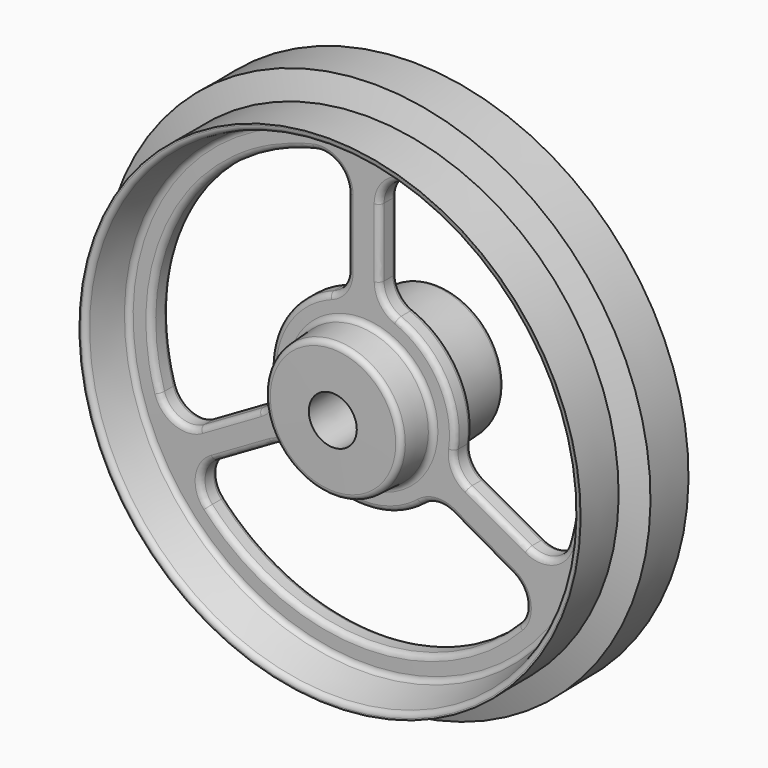
from build123d import *

# Parameters (mm, degrees)
F3_DEPTH = 43.6186672242
F4_R     = 2.54


with BuildPart() as f1:
    # F0 (on Right) → F1 (revolve)
    with BuildSketch(Plane.YZ):
        with BuildLine():
            Line((-17.1431349548, 28.9278083222), (-17.1431349548, 10.9819196094))
            Line((-17.1431349548, 10.9819196094), (43.1818650452, 10.9819196094))
            Line((43.1818650452, 10.9819196094), (43.1818650452, 28.867559352))
            ThreePointArc((43.1818650452, 28.867559352), (42.4756452655, 30.6250718281), (40.7496996094, 31.4052692856))
            Line((40.7496996094, 31.4052692856), (12.594030481, 32.601684317))
            ThreePointArc((12.594030481, 32.601684317), (10.8680848248, 33.3818817744), (10.1618650452, 35.1393942505))
            Line((10.1618650452, 35.1393942505), (10.1618650452, 115.7784299063))
            ThreePointArc((10.1618650452, 115.7784299063), (10.6173699596, 117.2298017531), (11.8205109018, 118.1606169002))
            Line((11.8205109018, 118.1606169002), (27.5388583799, 123.9760422684))
            ThreePointArc((27.5388583799, 123.9760422684), (28.7419993222, 124.9068574154), (29.1975042365, 126.3582292623))
            Line((29.1975042365, 126.3582292623), (29.1975042365, 127.2266535884))
            Line((29.1975042365, 127.2266535884), (6.9725042365, 127.2266535884))
            Line((6.9725042365, 127.2266535884), (2.6667747842, 115.951028812))
            Line((2.6667747842, 115.951028812), (-19.5582252158, 115.951028812))
            Line((-19.5582252158, 115.951028812), (-19.5582252158, 115.2566707518))
            ThreePointArc((-19.5582252158, 115.2566707518), (-19.0016386227, 113.6699536197), (-17.575806903, 112.7786266315))
            Line((-17.575806903, 112.7786266315), (-1.9805532676, 109.269557619))
            ThreePointArc((-1.9805532676, 109.269557619), (-0.5547215479, 108.3782306309), (0.0018650452, 106.7915134988))
            Line((0.0018650452, 106.7915134988), (0.0018650452, 34.8349003864))
            ThreePointArc((0.0018650452, 34.8349003864), (-0.6825103243, 33.1004675596), (-2.3668414357, 32.3006828484))
            Line((-2.3668414357, 32.3006828484), (-14.7744284739, 31.4620258603))
            ThreePointArc((-14.7744284739, 31.4620258603), (-16.4587595853, 30.662241149), (-17.1431349548, 28.9278083222))
        make_face()
    revolve(axis=Axis((0, -8.6872753461, -0.0663357208), (0, -0.9999708473, -0.0076357413)))

    # F2 (on Front) → F3 (cut, through all)
    with BuildSketch(Plane.XZ):
        with BuildLine():
            Line((-6.7658544631, 51.822418936), (-6.7658544631, 83.3901949943))
            ThreePointArc((-6.7658544631, 83.3901949943), (-11.5720090409, 93.33892378), (-22.3528157938, 95.7577110859))
            ThreePointArc((-22.3528157938, 95.7577110859), (-84.8589980062, 49.680358933), (-94.4432492338, -27.3799247713))
            ThreePointArc((-94.4432492338, -27.3799247713), (-86.9661995123, -35.6337295109), (-75.8589460274, -34.8210270811))
            Line((-75.8589460274, -34.8210270811), (-48.408480742, -18.8504932245))
            ThreePointArc((-48.408480742, -18.8504932245), (-43.3625739207, -13.4038718555), (-42.2241365486, -6.0669228754))
            ThreePointArc((-42.2241365486, -6.0669228754), (-36.7105113145, 21.7261045629), (-15.0000612074, 39.9334875039))
            ThreePointArc((-15.0000612074, 39.9334875039), (-9.0254144737, 44.5914291817), (-6.7658544631, 51.822418936))
        make_face()
        with BuildLine():
            ThreePointArc((23.8493413892, 95.3959984571), (12.9533792237, 93.0854213315), (8.0690974061, 83.0751990916))
            Line((8.0690974061, 83.0751990916), (8.0690974061, 51.3140057615))
            ThreePointArc((8.0690974061, 51.3140057615), (10.2381265661, 44.2155092188), (16.0043183773, 39.5417128325))
            ThreePointArc((16.0043183773, 39.5417128325), (37.0297436849, 21.1774253176), (42.1964618524, -6.2565060206))
            ThreePointArc((42.1964618524, -6.2565060206), (43.3372856677, -13.6718080208), (48.4641868849, -19.1493135334))
            Line((48.4641868849, -19.1493135334), (75.959996049, -34.8412705892))
            ThreePointArc((75.959996049, -34.8412705892), (87.0270006495, -35.5804792567), (94.4540776935, -27.3425458469))
            ThreePointArc((94.4540776935, -27.3425458469), (85.23562815, 49.0313705723), (23.8493413892, 95.3959984571))
        make_face()
        with BuildLine():
            ThreePointArc((-69.5086926909, -46.8883695864), (-75.6777297253, -55.9559683063), (-72.4837180262, -66.4477104755))
            ThreePointArc((-72.4837180262, -66.4477104755), (-0.8480583522, -98.3283702873), (71.3268296883, -67.68804158))
            ThreePointArc((71.3268296883, -67.68804158), (74.6879043591, -57.1559612965), (68.5212926465, -47.9802085739))
            Line((68.5212926465, -47.9802085739), (41.2527459246, -32.0486723221))
            ThreePointArc((41.2527459246, -32.0486723221), (33.8811048936, -30.3510231304), (26.851835465, -33.1461037319))
            ThreePointArc((26.851835465, -33.1461037319), (-0.5669770227, -42.6540009554), (-27.7233797542, -32.4206643278))
            ThreePointArc((-27.7233797542, -32.4206643278), (-34.8323278226, -29.4245938597), (-42.3636936899, -31.0955543799))
            Line((-42.3636936899, -31.0955543799), (-69.5086926909, -46.8883695864))
        make_face()
    extrude(amount=-F3_DEPTH, mode=Mode.SUBTRACT)

    # F4
    f4_edges = [f1.edges().sort_by_distance(p)[0] for p in [
        (0, 0.001865, 70.813207),
        (0, 0.53383, -34.83081),
        (0, 1.632682, -106.779032),
        (-0.848072, 1.503645, -98.32837),
        (74.687877, 1.156507, -57.155768),
        (54.887021, 0.826121, -40.014441),
        (33.881233, 0.580994, -30.351013),
        (-0.566984, 0.653341, -42.654001),
        (-34.832458, 0.574756, -29.424582),
        (-55.936194, 0.820304, -38.991963),
        (-75.677701, 1.147875, -55.95578),
        (-6.765854, 0.004444, 67.606307),
        (-11.572012, 0.007322, 93.338926),
        (-84.85933, 0.373377, 49.679791),
        (-86.966072, 0.991656, -35.633781),
        (-62.133715, 0.723623, -26.835761),
        (-43.362609, 0.450808, -13.403944),
        (-36.71062, 0.161702, 21.72592),
        (-9.025418, 0.00877, 44.591424),
        (8.069097, 0.005551, 67.194602),
        (10.238131, 0.010798, 44.215503),
        (37.029845, 0.165892, 21.177247),
        (43.337321, 0.453279, -13.67188),
        (62.212093, 0.725875, -26.995293),
        (87.026876, 0.991526, -35.58053),
        (85.235948, 0.378333, 49.030814),
        (12.953383, 0.008714, 93.085424),
        (0, 10.161865, 75.458912),
        (0, 11.928737, -115.609747),
        (0, 10.697295, -34.980114),
        (-36.710621, 10.321993, 21.72592),
        (-43.362609, 10.611576, -13.403943),
        (-62.133715, 10.884451, -26.835761),
        (-86.966072, 11.152474, -35.633781),
        (-84.859331, 10.53367, 49.67979),
        (-11.572012, 10.167326, 93.338926),
        (-6.765854, 10.164447, 67.606307),
        (-9.025418, 10.168781, 44.591424),
        (85.235949, 10.53863, 49.030813),
        (87.026876, 11.152342, -35.58053),
        (62.212093, 10.886703, -26.995293),
        (43.337321, 10.614051, -13.67188),
        (37.029846, 10.326191, 21.177247),
        (10.238131, 10.170813, 44.215503),
        (8.069097, 10.165556, 67.194602),
        (12.953383, 10.16872, 93.085424),
        (-55.936194, 10.981236, -38.991963),
        (-34.832458, 10.735732, -29.424582),
        (-0.566984, 10.814526, -42.654001),
        (33.881232, 10.741982, -30.351013),
        (54.887021, 10.987063, -40.014441),
        (74.687877, 11.31746, -57.155768),
        (-0.848072, 11.664829, -98.32837),
        (-75.677701, 11.30882, -55.95578),
    ]]
    fillet(f4_edges, radius=F4_R)


solid = f1.part
